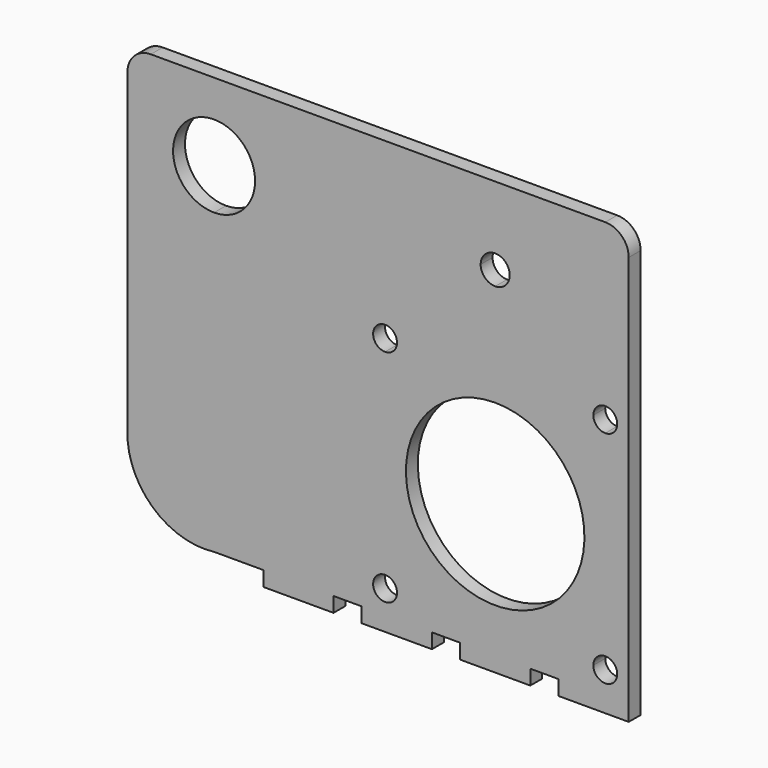
from build123d import *

# Parameters (mm, degrees)
F0_W     = 15
F0_H     = 3.175
F0_W_2   = 7.5
F1_DEPTH = 3.175


# Not quite as in the source:
# - a feature names something its author has since deleted; it is built from what else it names


with BuildPart() as f1:
    # F0 (on Front) → F1 (new body)
    with BuildSketch(Plane.XZ):
        Polygon((0, 28.5), (-28.5, 28.5), (-28.5, -28.5), (-13.5, -28.5), (-7.5, -28.5), (0, -28.5), (7.5, -28.5), (13.5, -28.5), (28.5, -28.5), (28.5, 23.5), (28.5, 28.5), (23.5, 28.5), align=None)
        with BuildLine():
            Line((-20.95, 23.5), (0, 23.5))
            Line((0, 23.5), (20.95, 23.5))
            ThreePointArc((20.95, 23.5), (23.5, 26.05), (26.05, 23.5))
            ThreePointArc((26.05, 23.5), (25.303122292, 21.696877708), (23.5, 20.95))
            Line((23.5, 20.95), (23.5, -20.95))
            ThreePointArc((23.5, -20.95), (25.303122292, -21.696877708), (26.05, -23.5))
            ThreePointArc((26.05, -23.5), (23.5, -26.05), (20.95, -23.5))
            Line((20.95, -23.5), (-20.95, -23.5))
            ThreePointArc((-20.95, -23.5), (-25.303122292, -25.303122292), (-23.5, -20.95))
            Line((-23.5, -20.95), (-23.5, 20.95))
            ThreePointArc((-23.5, 20.95), (-25.303122292, 25.303122292), (-20.95, 23.5))
        make_face(mode=Mode.SUBTRACT)
        with BuildLine():
            Line((-28.5, -28.5), (-28.5, 28.5))
            Line((-28.5, 28.5), (-28.5, 44))
            Line((-28.5, 44), (-51.25, 44))
            ThreePointArc((-51.25, 44), (-53.8128156646, 37.8128156646), (-60, 35.25))
            Line((-60, 35.25), (-60, -28.5))
            Line((-60, -28.5), (-49.5, -28.5))
            Line((-49.5, -28.5), (-34.5, -28.5))
            Line((-34.5, -28.5), (-28.5, -28.5))
        make_face()
        with BuildLine():
            Line((20.95, 23.5), (0, 23.5))
            Line((0, 23.5), (-20.95, 23.5))
            ThreePointArc((-20.95, 23.5), (-21.696877708, 21.696877708), (-23.5, 20.95))
            Line((-23.5, 20.95), (-23.5, -20.95))
            ThreePointArc((-23.5, -20.95), (-21.696877708, -21.696877708), (-20.95, -23.5))
            Line((-20.95, -23.5), (20.95, -23.5))
            ThreePointArc((20.95, -23.5), (21.696877708, -21.696877708), (23.5, -20.95))
            Line((23.5, -20.95), (23.5, 20.95))
            ThreePointArc((23.5, 20.95), (21.696877708, 21.696877708), (20.95, 23.5))
        make_face()
        with BuildLine():
            ThreePointArc((19.05, 0), (-13.4703841816, -13.4703841816), (0, 19.05))
            ThreePointArc((0, 19.05), (13.4703841816, 13.4703841816), (19.05, 0))
        make_face(mode=Mode.SUBTRACT)
        with BuildLine():
            Line((-51.25, 44), (-28.5, 44))
            Line((-28.5, 44), (-28.5, 60.5991594493))
            Line((-28.5, 60.5991594493), (-73.5, 60.5991594493))
            ThreePointArc((-73.5, 60.5991594493), (-77.0355339059, 59.1346933553), (-78.5, 55.5991594493))
            Line((-78.5, 55.5991594493), (-78.5, -11.5))
            ThreePointArc((-78.5, -11.5), (-73.1911039749, -24.2888484433), (-60, -28.5))
            Line((-60, -28.5), (-60, 35.25))
            ThreePointArc((-60, 35.25), (-66.1871843354, 50.1871843354), (-51.25, 44))
        make_face()
        with BuildLine():
            Line((0, 40.9), (0, 28.5))
            Line((0, 28.5), (23.5, 28.5))
            Line((23.5, 28.5), (28.5, 28.5))
            Line((28.5, 28.5), (28.5, 55.5991594493))
            ThreePointArc((28.5, 55.5991594493), (27.0355339059, 59.1346933553), (23.5, 60.5991594493))
            Line((23.5, 60.5991594493), (-28.5, 60.5991594493))
            Line((-28.5, 60.5991594493), (-28.5, 44))
            Line((-28.5, 44), (-3.1, 44))
            ThreePointArc((-3.1, 44), (0, 47.1), (3.1, 44))
            ThreePointArc((3.1, 44), (2.1920310217, 41.8079689783), (0, 40.9))
        make_face()
        with BuildLine():
            Line((-28.5, 44), (-28.5, 28.5))
            Line((-28.5, 28.5), (0, 28.5))
            Line((0, 28.5), (0, 40.9))
            ThreePointArc((0, 40.9), (-2.1920310217, 41.8079689783), (-3.1, 44))
            Line((-3.1, 44), (-28.5, 44))
        make_face()
        with Locations((21, -30.0875)):
            Rectangle(F0_W, F0_H)
        with Locations((-21, -30.0875)):
            Rectangle(F0_W, F0_H)
        with Locations((-42, -30.0875)):
            Rectangle(F0_W, F0_H)
        with Locations((3.75, -30.0875)):
            Rectangle(F0_W_2, F0_H)
        with Locations((-3.75, -30.0875)):
            Rectangle(F0_W_2, F0_H)
    extrude(amount=F1_DEPTH)


solid = f1.part
